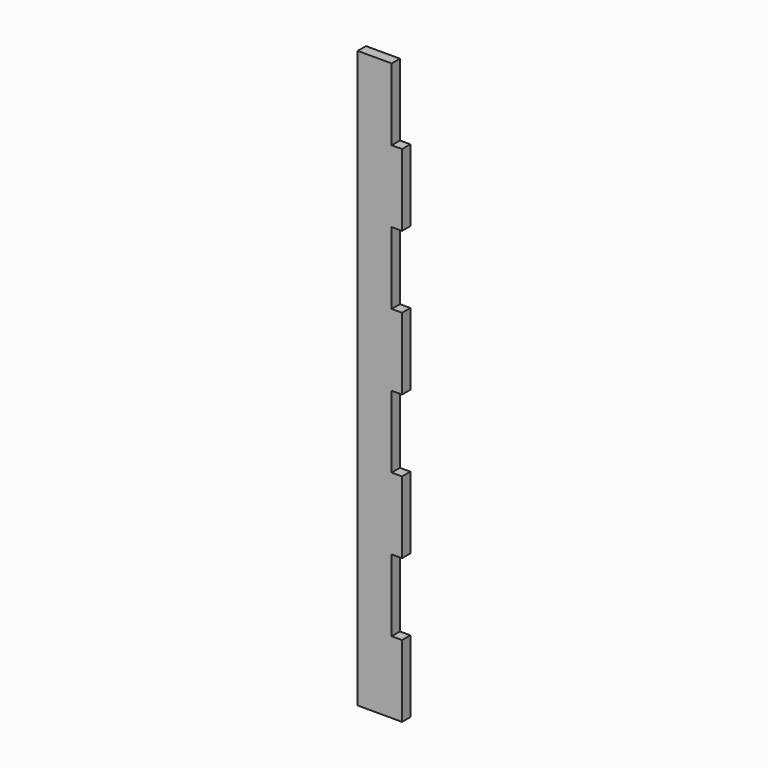
from build123d import *

# Parameters (mm, degrees)
F1_DEPTH = 18


# Not quite as in the source:
# - a feature names something its author has since deleted; it is built from what else it names


with BuildPart() as f1:
    # F0 (on Front) → F1 (new body)
    with BuildSketch(Plane.XZ):
        Polygon((0, 1000), (0, 0), (77, 0), (77, 125), (59, 125), (59, 250), (77, 250), (77, 375), (59, 375), (59, 500), (77, 500), (77, 625), (59, 625), (59, 750), (77, 750), (77, 875), (59, 875), (59, 1000), align=None)
    extrude(amount=F1_DEPTH)


solid = f1.part
